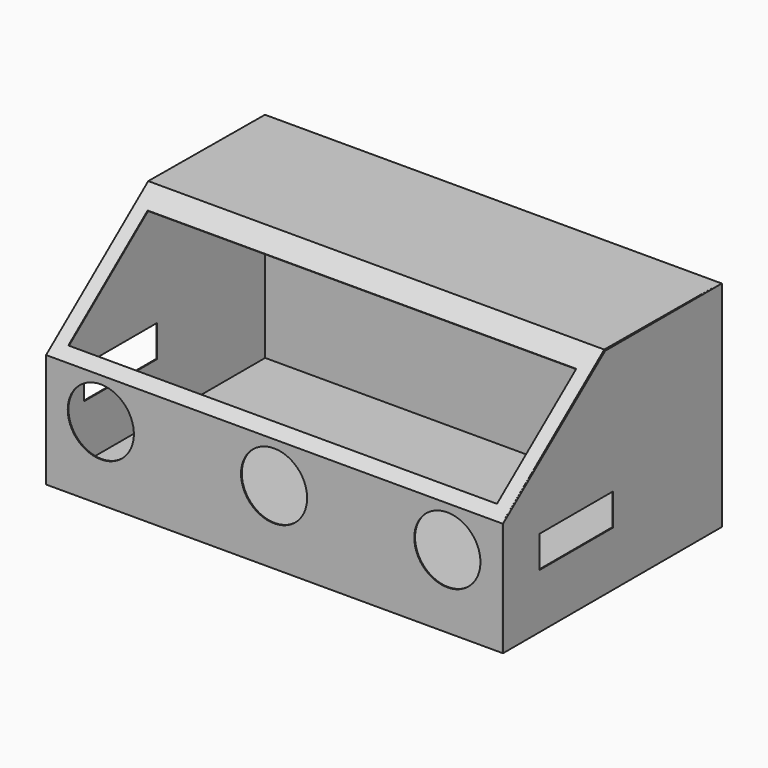
from build123d import *

# Parameters (mm, degrees)
F2_DEPTH = 1000
F3_W     = 940
F3_H     = 277.328980073
F4_DEPTH = 5
F6_D     = 145
F6_DEPTH = 4
F6_TIP   = 43.5623948795
F1_W     = 200
F1_H     = 70
F7_DEPTH = 2
F8_W     = 201.8966459586
F8_H     = 70
F9_DEPTH = 2


with BuildPart() as f2:
    # F1 (on Right) → F2 (new body)
    with BuildSketch(Plane.YZ):
        Polygon((-288.5542339748, 27.2076225815), (-288.5542339748, -222.7923774185), (311.4457660252, -222.7923774185), (311.4457660252, 247.2076225815), (-8.5542339748, 249.2076225815), align=None)
        Polygon((-286.5542339748, 26.2409870095), (-7.8630740966, 247.2032637701), (309.4457660252, 245.2200835194), (309.4457660252, -220.7923774185), (-286.5542339748, -220.7923774185), align=None, mode=Mode.SUBTRACT)
    extrude(amount=F2_DEPTH)

    # F3 (on face) → F4 (cut)
    with BuildSketch(Plane(origin=(0, -124.6227615588, 157.1818614256), x_dir=(1, 0, 0), z_dir=(0, -0.6212762255, 0.7835916358))):
        with Locations((500, -40.5407451073)):
            Rectangle(F3_W, F3_H)
    extrude(amount=-F4_DEPTH, mode=Mode.SUBTRACT)

    # F6
    with Locations(Plane.XZ.offset(288.5542339748)):
        with Locations((120, -62.7923774185), (500, -62.7923774185), (880, -62.7923774185)):
            Hole(F6_D / 2, depth=F6_DEPTH)
            with Locations((0, 0, -(F6_DEPTH + F6_TIP / 2))):  # 118° drill point
                Cone(0, F6_D / 2, F6_TIP, mode=Mode.SUBTRACT)

    # F1 (on Right) → F7 (join)
    with BuildSketch(Plane.YZ):
        Polygon((309.4457660252, 245.2200835194), (-7.8630740966, 247.2032637701), (-286.5542339748, 26.2409870095), (-286.5542339748, -220.7923774185), (309.4457660252, -220.7923774185), align=None)
        with Locations((-86.5542339748, -67.7923774185)):
            Rectangle(F1_W, F1_H, mode=Mode.SUBTRACT)
    extrude(amount=F7_DEPTH)

    # F8 (on face) → F9 (join)
    with BuildSketch(Plane.YZ.offset(1000)):
        Polygon((-288.4508799334, 27.2547214809), (-288.4508799334, -222.7452785191), (311.5491200666, -222.7452785191), (311.5491200666, 247.2547214809), (-8.4508799334, 247.2547214809), align=None)
        with Locations((-87.5025569541, -67.7452785191)):
            Rectangle(F8_W, F8_H, mode=Mode.SUBTRACT)
    extrude(amount=F9_DEPTH)


solid = f2.part
